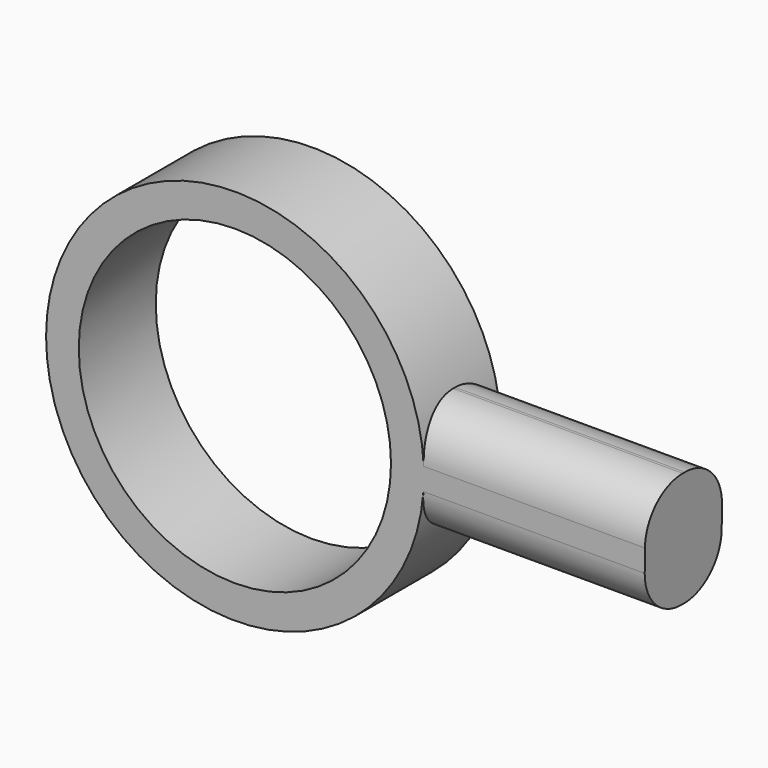
from build123d import *

# Parameters (mm, degrees)
F1_DEPTH     = 14.0906665474
F3_D         = 45.72
F4_R         = 6.858
F5_T4_DEPTH  = 103.1253973126
F5_S5_R      = 27.6648668559
F5_T6_DEPTH  = 53
F5_T10_DEPTH = 103.1253973126
F5_S11_R     = 27.6648668559
F5_T12_DEPTH = 53


# Not quite as in the source:
# - a fillet or chamfer that OpenCascade refuses, or shapes differently, is made with other operations: its cross-section is extruded or revolved along the edge and cut away or added


with BuildPart() as f1:
    # F0 (on Front) → F1 (new body)
    with BuildSketch(Plane.XZ):
        with BuildLine():
            ThreePointArc((26.2165333562, -8.9155114296), (27.3140546761, -4.5315667493), (27.6831785203, -0.0274273648))
            ThreePointArc((27.6831785203, -0.0274273648), (27.3786909177, 4.0657993906), (26.4719306688, 8.0689236483))
            Line((26.4719306688, 8.0689236483), (-26.4353073399, 8.0689236483))
            Line((-26.4353073399, 8.0689236483), (-26.4353073399, -8.1237783779))
            ThreePointArc((-26.4353073399, -8.1237783779), (-26.3105848654, -8.5206049607), (-26.1799100273, -8.9155114296))
            Line((-26.1799100273, -8.9155114296), (26.2165333562, -8.9155114296))
        make_face()
        with BuildLine():
            ThreePointArc((26.4719306688, 8.0689236483), (27.3786909177, 4.0657993906), (27.6831785203, -0.0274273648))
            ThreePointArc((27.6831785203, -0.0274273648), (27.3140546761, -4.5315667493), (26.2165333562, -8.9155114296))
            Line((26.2165333562, -8.9155114296), (59.9537639373, -8.9155114296))
            Line((59.9537639373, -8.9155114296), (60.1102084538, 8.0689236483))
            Line((60.1102084538, 8.0689236483), (26.4719306688, 8.0689236483))
        make_face()
        with BuildLine():
            Line((-26.4353073399, 8.0689236483), (26.4719306688, 8.0689236483))
            ThreePointArc((26.4719306688, 8.0689236483), (0.0183116645, 27.6374394911), (-26.4353073399, 8.0689236483))
        make_face()
        with BuildLine():
            ThreePointArc((-26.1799100273, -8.9155114296), (0.0183116645, -27.6922942207), (26.2165333562, -8.9155114296))
            Line((26.2165333562, -8.9155114296), (-26.1799100273, -8.9155114296))
        make_face()
        with BuildLine():
            Line((-26.4353073399, -8.1237783779), (-26.4353073399, 8.0689236483))
            ThreePointArc((-26.4353073399, 8.0689236483), (-27.6465551914, -0.0274273648), (-26.4353073399, -8.1237783779))
        make_face()
        with BuildLine():
            Line((-26.4353073399, -8.9155114296), (-26.1799100273, -8.9155114296))
            ThreePointArc((-26.1799100273, -8.9155114296), (-26.3105848654, -8.5206049607), (-26.4353073399, -8.1237783779))
            Line((-26.4353073399, -8.1237783779), (-26.4353073399, -8.9155114296))
        make_face()
    extrude(amount=F1_DEPTH)

    # F3 (through all)
    with Locations(Plane(origin=(0, 0, 0), x_dir=(1, 0, 0), z_dir=(0, 1, 0))):
        with Locations((0, 0)):
            Hole(F3_D / 2)

    # F4
    f4_edges = [f1.edges().sort_by_distance(p)[0] for p in [
        (43.085149, -14.090667, -8.915511),
        (43.085149, 0, -8.915511),
        (43.29107, -14.090667, 8.068924),
        (43.29107, 0, 8.068924),
    ]]
    fillet(f4_edges, radius=F4_R)

    # F5: fillet of radius 6.858 on 2 edges, made by hand


with BuildPart() as f5_tool2:
    # F5_s3 → F5_t4 (new body)
    with BuildSketch(Plane.YZ.offset(-43.5803073399)):
        with BuildLine():
            ThreePointArc((-14.0906665474, -2.0575114296), (-12.0820048528, -6.906849735), (-7.2326665474, -8.9155114296))
            Line((-7.2326665474, -8.9155114296), (-14.0906665474, -8.9155114296))
            Line((-14.0906665474, -8.9155114296), (-14.0906665474, -2.0575114296))
        make_face()
    extrude(amount=F5_T4_DEPTH)

    # F5_s5 → F5_t6 (cut, symmetric)
    with BuildSketch(Plane.XZ.offset(10.7)):
        with Locations((0.0183116645, -0.0274273648)):
            Circle(F5_S5_R)
    extrude(amount=F5_T6_DEPTH, both=True, mode=Mode.SUBTRACT)


with BuildPart() as f1_1:
    add(f1.part)

    # F5_t1: cut F5_tool2
    add(f5_tool2.part, mode=Mode.SUBTRACT)


with BuildPart() as f5_tool8:
    # F5_s9 → F5_t10 (new body)
    with BuildSketch(Plane.YZ.offset(-43.5803073399)):
        with BuildLine():
            ThreePointArc((0, -2.0575114296), (-2.0086616946, -6.906849735), (-6.858, -8.9155114296))
            Line((-6.858, -8.9155114296), (0, -8.9155114296))
            Line((0, -8.9155114296), (0, -2.0575114296))
        make_face()
    extrude(amount=F5_T10_DEPTH)

    # F5_s11 → F5_t12 (cut, symmetric)
    with BuildSketch(Plane.XZ.offset(3.4)):
        with Locations((0.0183116645, -0.0274273648)):
            Circle(F5_S11_R)
    extrude(amount=F5_T12_DEPTH, both=True, mode=Mode.SUBTRACT)


with BuildPart() as f1_2:
    add(f1_1.part)

    # F5_t7: cut F5_tool8
    add(f5_tool8.part, mode=Mode.SUBTRACT)


solid = f1_2.part
